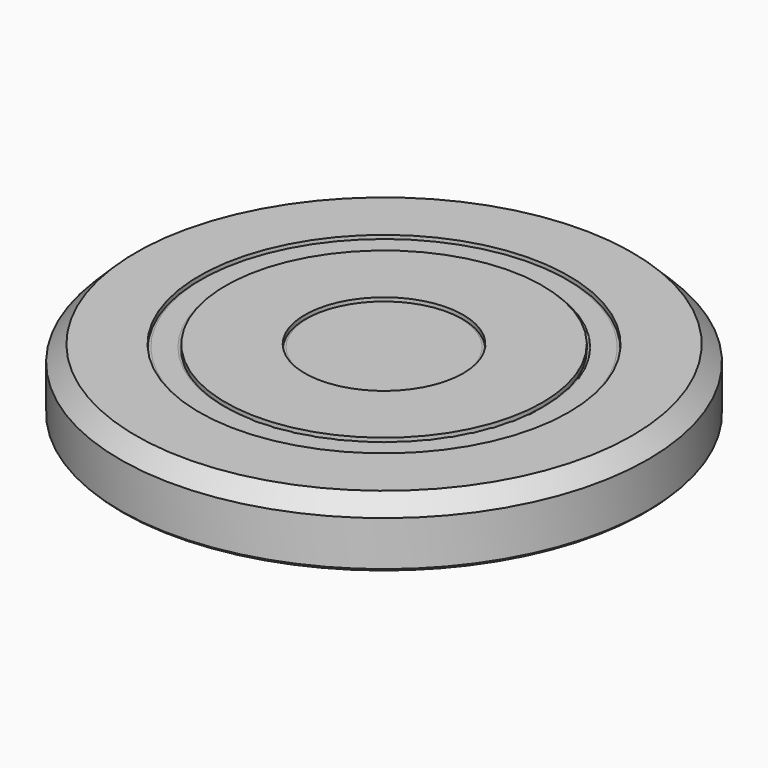
from build123d import *
from build123d import SkipClean  # not in build123d's __all__

# Parameters (mm, degrees)
F0_R      = 50
F1_DEPTH  = 12
F2_SIZE   = 3
F3_SIZE   = 0.5
F4_R      = 35
F4_R_2    = 30
F4_R_3    = 15
F5_DEPTH  = 3
F6_R      = 35
F6_R_2    = 30
F7_DEPTH  = 2.5
F6_R_3    = 15
F8_R      = 0.5
F9_R      = 0.5
F10_T     = -1
F11_W     = 17.1537045389
F11_H     = 3.4956783056
F12_DEPTH = 1.5
F13_R     = 4
F14_DEPTH = 0.7
F15_R     = 2
F16_DEPTH = 8.301


with BuildPart() as f1:
    # F0 (on Top) → F1 (new body)
    with BuildSketch(Plane.XY):
        Circle(F0_R)
    extrude(amount=F1_DEPTH)

    # F2
    f2_edges = [f1.edges().sort_by_distance(p)[0] for p in [
        (-50, 0, 12),
    ]]
    chamfer(f2_edges, length=F2_SIZE)

    # F3
    f3_edges = [f1.edges().sort_by_distance(p)[0] for p in [
        (-50, 0, 0),
    ]]
    chamfer(f3_edges, length=F3_SIZE)

    # F4 (on face) → F5 (cut)
    with BuildSketch(Plane.XY.offset(12)):
        Circle(F4_R)
        Circle(F4_R_2, mode=Mode.SUBTRACT)
        Circle(F4_R_3)
    extrude(amount=-F5_DEPTH, mode=Mode.SUBTRACT)

    # F10
    f10_openings = [f1.faces().sort_by_distance(p)[0] for p in [
        (0, 0, 0),
    ]]
    offset(amount=F10_T, openings=f10_openings, kind=Kind.INTERSECTION)

    # F11 (on face) → F12 (cut)
    with BuildSketch(Plane(origin=(0, 0, 0), x_dir=(1, 0, 0), z_dir=(0, 0, -1))):
        with Locations((0, -48.7780682743)):
            Rectangle(F11_W, F11_H)
    extrude(amount=-F12_DEPTH, mode=Mode.SUBTRACT)

    # F13 (on face) → F14 (cut)
    with BuildSketch(Plane.XY.offset(9)):
        Circle(F13_R)
    extrude(amount=-F14_DEPTH, mode=Mode.SUBTRACT)

    # F15 (on face) → F16 (cut, through all)
    with BuildSketch(Plane.XY.offset(8.3)):
        Circle(F15_R)
    extrude(amount=-F16_DEPTH, mode=Mode.SUBTRACT)

    # F18 (on face) → F19 (revolve, cut)
    with BuildSketch(Plane(origin=(8.5768522695, 0, 0), x_dir=(0, -1, 0), z_dir=(-1, 0, 0))):
        Polygon((-47.3146960518, 0), (-48.2435239711, 0.9142135624), (-48.2435239711, 0), align=None)
    with SkipClean():  # cleaning this boolean's faces spoils the solid; the shape is the same uncleaned
        revolve(axis=Axis((0, 0, 0.4506437108), (0, 0, -1)), mode=Mode.SUBTRACT)


with BuildPart() as f7:
    # F6 (on face) → F7 (new body)
    with BuildSketch(Plane.XY.offset(9)):
        Circle(F6_R)
        Circle(F6_R_2, mode=Mode.SUBTRACT)
    extrude(amount=F7_DEPTH)

    # F8
    f8_edges = [f7.edges().sort_by_distance(p)[0] for p in [
        (-35, 0, 11.5),
        (-30, 0, 11.5),
    ]]
    fillet(f8_edges, radius=F8_R)


with BuildPart() as f7b:
    # F6 (on face) → F7, piece 2 (new body)
    with BuildSketch(Plane.XY.offset(9)):
        Circle(F6_R_3)
    extrude(amount=F7_DEPTH)

    # F9
    f9_edges = [f7b.edges().sort_by_distance(p)[0] for p in [
        (-15, 0, 11.5),
    ]]
    fillet(f9_edges, radius=F9_R)


solid = Compound([f1.part, f7.part, f7b.part])
